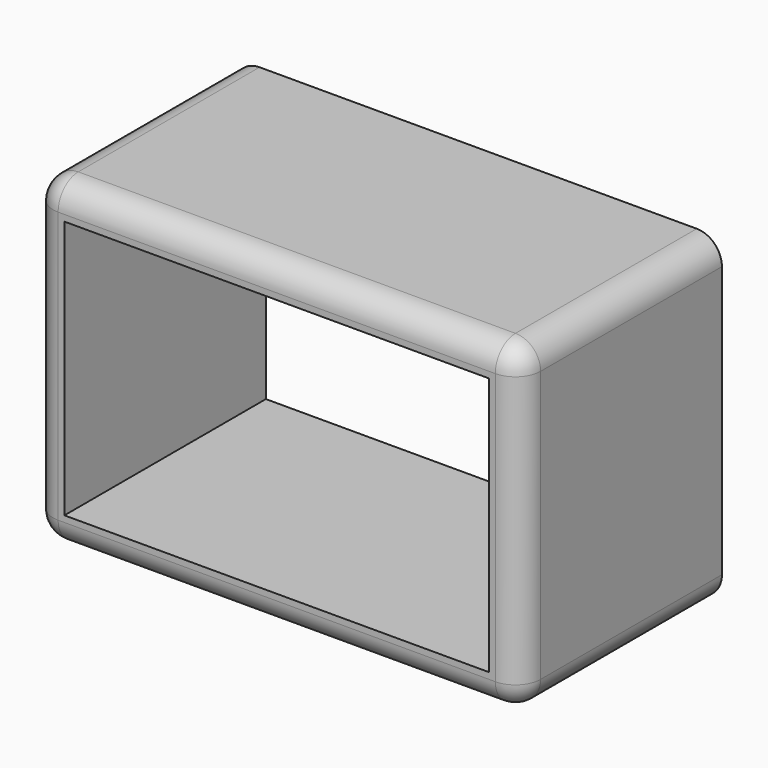
from build123d import *

# Parameters (mm, degrees)
F1_W         = 98.3519479632
F1_H         = 64.8710429668
F1_W_2       = 85.651949048
F1_H_2       = 52.1710440516
F2_DEPTH     = 50.8
F3_R         = 5.08
F4_T1_DEPTH  = 58.42
F4_S5_W      = 5.08
F4_S5_H      = 5.08
F4_T6_DEPTH  = 5.08
F4_S11_W     = 5.08
F4_S11_H     = 5.08
F4_T12_DEPTH = 5.08
F4_S17_W     = 5.08
F4_S17_H     = 5.08
F4_T18_DEPTH = 5.08
F5_T1_DEPTH  = 58.42
F5_S5_W      = 5.08
F5_S5_H      = 5.08
F5_T6_DEPTH  = 5.08


# Not quite as in the source:
# - a fillet or chamfer that OpenCascade refuses, or shapes differently, is made with other operations: its cross-section is extruded or revolved along the edge and cut away or added


with BuildPart() as f2:
    # F1 (on face) → F2 (new body)
    with BuildSketch(Plane.XZ):
        with Locations((0.1114979386, 7.887352258)):
            Rectangle(F1_W, F1_H)
        with Locations((0.1114979386, 7.887352258)):
            Rectangle(F1_W_2, F1_H_2, mode=Mode.SUBTRACT)
    extrude(amount=F2_DEPTH)

    # F3
    f3_edges = [f2.edges().sort_by_distance(p)[0] for p in [
        (0.111498, -50.8, 40.322874),
        (49.287472, -50.8, 7.887352),
        (0.111498, -50.8, -24.548169),
        (-49.064476, -50.8, 7.887352),
    ]]
    fillet(f3_edges, radius=F3_R)

    # F4: fillet of radius 5.08 on 3 edges, made by hand

    # F4_s2 → F4_t1 (cut)
    with BuildSketch(Plane.XZ.offset(-12.7)):
        with BuildLine():
            ThreePointArc((44.2074719203, 40.3228737414), (47.7995743687, 38.8349761898), (49.2874719203, 35.2428737414))
            Line((49.2874719203, 35.2428737414), (49.2874719203, 40.3228737414))
            Line((49.2874719203, 40.3228737414), (44.2074719203, 40.3228737414))
        make_face()
        with BuildLine():
            ThreePointArc((49.2874719203, -19.4681692255), (47.7995743687, -23.0602716739), (44.2074719203, -24.5481692255))
            Line((44.2074719203, -24.5481692255), (49.2874719203, -24.5481692255))
            Line((49.2874719203, -24.5481692255), (49.2874719203, -19.4681692255))
        make_face()
        with BuildLine():
            ThreePointArc((-49.064476043, -19.4681692255), (-47.5765784914, -23.0602716739), (-43.984476043, -24.5481692255))
            Line((-43.984476043, -24.5481692255), (-49.064476043, -24.5481692255))
            Line((-49.064476043, -24.5481692255), (-49.064476043, -19.4681692255))
        make_face()
    extrude(amount=F4_T1_DEPTH, mode=Mode.SUBTRACT)


with BuildPart() as f4_tool4:
    # F4_s5 → F4_t6 (new body)
    with BuildSketch(Plane.YZ.offset(-43.984476043)):
        with Locations((-48.26, -22.0081692255)):
            Rectangle(F4_S5_W, F4_S5_H)
    extrude(amount=-F4_T6_DEPTH)

    # F4_s7 → F4_t8 (revolve, cut)
    with BuildSketch(Plane(origin=(-43.984476043, -45.72, -19.4681692255), x_dir=(0, 0.7071067812, 0.7071067812), z_dir=(0, -0.7071067812, 0.7071067812))):
        with BuildLine():
            ThreePointArc((0, -5.08), (5.08, 0), (0, 5.08))
            Line((0, 5.08), (0, -5.08))
        make_face()
    revolve(axis=Axis((-43.984476043, -45.72, -19.4681692255), (-1, 0, 0)), mode=Mode.SUBTRACT)


with BuildPart() as f2_1:
    add(f2.part)

    # F4_t3: cut F4_tool4
    add(f4_tool4.part, mode=Mode.SUBTRACT)


with BuildPart() as f4_tool10:
    # F4_s11 → F4_t12 (new body)
    with BuildSketch(Plane.YZ.offset(44.2074719203)):
        with Locations((-48.26, -22.0081692255)):
            Rectangle(F4_S11_W, F4_S11_H)
    extrude(amount=F4_T12_DEPTH)

    # F4_s13 → F4_t14 (revolve, cut)
    with BuildSketch(Plane(origin=(44.2074719203, -45.72, -19.4681692255), x_dir=(0, 0.7071067812, 0.7071067812), z_dir=(0, 0.7071067812, -0.7071067812))):
        with BuildLine():
            ThreePointArc((0, -5.08), (5.08, 0), (0, 5.08))
            Line((0, 5.08), (0, -5.08))
        make_face()
    revolve(axis=Axis((44.2074719203, -45.72, -19.4681692255), (1, 0, 0)), mode=Mode.SUBTRACT)


with BuildPart() as f2_2:
    add(f2_1.part)

    # F4_t9: cut F4_tool10
    add(f4_tool10.part, mode=Mode.SUBTRACT)


with BuildPart() as f4_tool16:
    # F4_s17 → F4_t18 (new body)
    with BuildSketch(Plane.XY.offset(35.2428737414)):
        with Locations((46.7474719203, -48.26)):
            Rectangle(F4_S17_W, F4_S17_H)
    extrude(amount=F4_T18_DEPTH)

    # F4_s19 → F4_t20 (revolve, cut)
    with BuildSketch(Plane(origin=(44.2074719203, -45.72, 35.2428737414), x_dir=(-0.7071067812, 0.7071067812, 0), z_dir=(0.7071067812, 0.7071067812, 0))):
        with BuildLine():
            ThreePointArc((0, -5.08), (5.08, 0), (0, 5.08))
            Line((0, 5.08), (0, -5.08))
        make_face()
    revolve(axis=Axis((44.2074719203, -45.72, 35.2428737414), (0, 0, 1)), mode=Mode.SUBTRACT)


with BuildPart() as f2_3:
    add(f2_2.part)

    # F4_t15: cut F4_tool16
    add(f4_tool16.part, mode=Mode.SUBTRACT)

    # F5: fillet of radius 5.08 on 1 edges, made by hand

    # F5_s2 → F5_t1 (cut)
    with BuildSketch(Plane.XZ.offset(-12.7)):
        with BuildLine():
            ThreePointArc((-43.984476043, 40.3228737414), (-47.5765784914, 38.8349761898), (-49.064476043, 35.2428737414))
            Line((-49.064476043, 35.2428737414), (-49.064476043, 40.3228737414))
            Line((-49.064476043, 40.3228737414), (-43.984476043, 40.3228737414))
        make_face()
    extrude(amount=F5_T1_DEPTH, mode=Mode.SUBTRACT)


with BuildPart() as f5_tool4:
    # F5_s5 → F5_t6 (new body)
    with BuildSketch(Plane.XY.offset(35.2428737414)):
        with Locations((-46.524476043, -48.26)):
            Rectangle(F5_S5_W, F5_S5_H)
    extrude(amount=F5_T6_DEPTH)

    # F5_s7 → F5_t8 (revolve, cut)
    with BuildSketch(Plane(origin=(-43.984476043, -45.72, 35.2428737414), x_dir=(0.7071067812, 0.7071067812, 0), z_dir=(0.7071067812, -0.7071067812, 0))):
        with BuildLine():
            ThreePointArc((0, -5.08), (5.08, 0), (0, 5.08))
            Line((0, 5.08), (0, -5.08))
        make_face()
    revolve(axis=Axis((-43.984476043, -45.72, 35.2428737414), (0, 0, 1)), mode=Mode.SUBTRACT)


with BuildPart() as f2_4:
    add(f2_3.part)

    # F5_t3: cut F5_tool4
    add(f5_tool4.part, mode=Mode.SUBTRACT)


solid = f2_4.part
